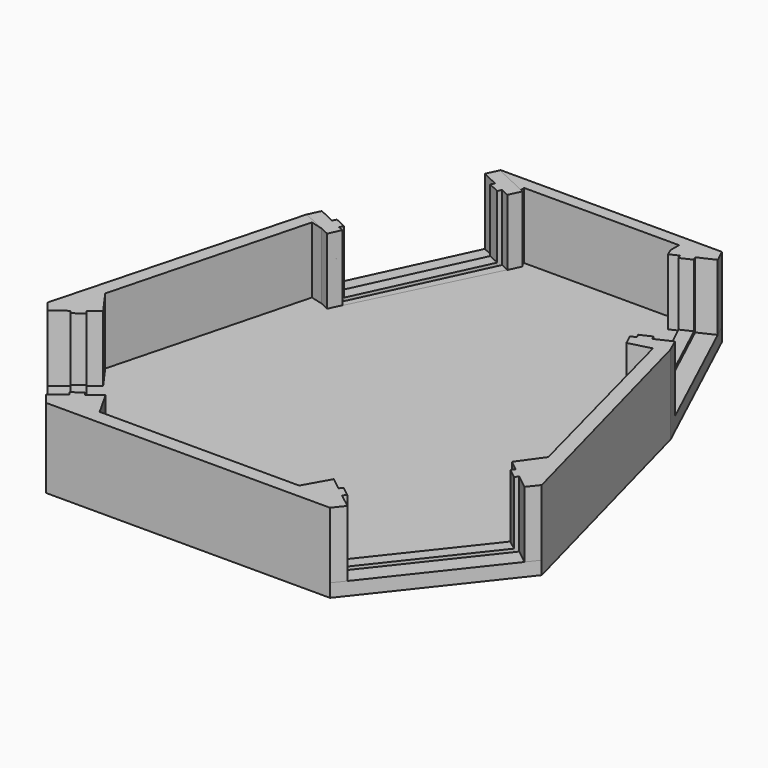
from build123d import *

# Parameters (mm, degrees)
F2_DEPTH  = 3
F4_DEPTH  = 0.7
F6_DEPTH  = 15
F7_DEPTH  = 0.7
F10_DEPTH = 15
F12_DEPTH = 3


with BuildPart() as f2:
    # F1 (on Top) → F2 (new body)
    with BuildSketch(Plane.XY):
        Polygon((25.0866528437, 0), (0, 0), (-25.0866528437, 0), (-41.3574559207, -34.8928498009), (-56.0353445751, -89.767503729), (-32.1974300433, -120), (0, -120), (32.1974300433, -120), (56.0353445751, -89.767503729), (41.3574559207, -34.8928498009), align=None)
    extrude(amount=-F2_DEPTH)

    # F3 (on face) → F4 (join)
    with BuildSketch(Plane.XY):
        Polygon((-33.371197317, -34.0930538801), (-20.5658639862, -6.6319279329), (-23.1035257899, -5.4485968), (-35.9088591207, -32.9097227472), align=None)
        Polygon((-50.2771969311, -90.448485161), (-31.5164486113, -114.2418523561), (-29.3177216098, -112.5081858447), (-48.0784699296, -88.7148186496), align=None)
        Polygon((20.5658639862, -6.6319279329), (33.371197317, -34.0930538801), (35.9088591207, -32.9097227472), (23.1035257899, -5.4485968), align=None)
        Polygon((29.3177216098, -112.5081858447), (31.5164486113, -114.2418523561), (50.2771969311, -90.448485161), (48.0784699296, -88.7148186496), align=None)
    extrude(amount=F4_DEPTH)

    # F5 (on face) → F6 (join)
    with BuildSketch(Plane.XY):
        Polygon((-23.1035257899, -5.4485968), (-20.5658639862, -6.6319279329), (-20.1643766376, -5.7709355352), (-18.2344874915, -6.6708576234), (-17.5556015009, -5.2149819182), (-17.5556015009, -2.7421381998), (0, -2.7421381998), (17.5556015009, -2.7421381998), (17.5556015009, -5.2149819182), (18.2344874915, -6.6708576234), (20.1643766376, -5.7709355352), (20.5658639862, -6.6319279329), (23.1035257899, -5.4485968), (22.7020384413, -4.5876044023), (26.4179003681, -2.8548695292), (25.0866528437, 0), (0, 0), (-25.0866528437, 0), (-26.4179003681, -2.8548695292), (-22.7020384413, -4.5876044023), align=None)
        Polygon((-33.7726846656, -34.9540462778), (-33.371197317, -34.0930538801), (-35.9088591207, -32.9097227472), (-36.3103464693, -33.7707151449), (-40.0262083962, -32.0379802717), (-41.3574559207, -34.8928498009), (-56.0353445751, -89.767503729), (-54.0849697497, -92.2410716057), (-50.8654052118, -89.7024884997), (-50.2771969311, -90.448485161), (-48.0784699296, -88.7148186496), (-48.6666782103, -87.9688219883), (-46.3434113852, -86.13695751), (-50.2389003724, -80.6826406293), (-38.6780583256, -36.5412120318), (-33.6958403856, -37.8460776983), (-32.6018529506, -35.5000140729), align=None)
        Polygon((-29.3177216098, -112.5081858447), (-31.5164486113, -114.2418523561), (-30.9282403307, -114.9878490173), (-34.1478048686, -117.5264321233), (-32.1974300433, -120), (0, -120), (32.1974300433, -120), (34.1478048686, -117.5264321233), (30.9282403307, -114.9878490173), (31.5164486113, -114.2418523561), (29.3177216098, -112.5081858447), (28.7295133292, -113.2541825059), (25.8780409714, -111.0058351069), (22.6252728403, -116.7735089854), (0, -116.7735089854), (-22.6252728403, -116.7735089854), (-25.8780409714, -111.0058351069), (-28.7295133292, -113.2541825059), align=None)
        Polygon((36.3103464693, -33.7707151449), (35.9088591207, -32.9097227472), (33.371197317, -34.0930538801), (33.7726846656, -34.9540462778), (32.6018529506, -35.5000140729), (33.6958403856, -37.8460776983), (38.6780583256, -36.5412120318), (50.2389003724, -80.6826406293), (46.3434113852, -86.13695751), (48.6666782103, -87.9688219883), (48.0784699296, -88.7148186496), (50.2771969311, -90.448485161), (50.8654052118, -89.7024884997), (54.0849697497, -92.2410716057), (56.0353445751, -89.767503729), (41.3574559207, -34.8928498009), (40.0262083962, -32.0379802717), align=None)
    extrude(amount=F6_DEPTH)


with BuildPart() as f7:
    # F3 (on face) → F7 (new body)
    with BuildSketch(Plane.XY):
        Polygon((-33.371197317, -34.0930538801), (-20.5658639862, -6.6319279329), (-23.1035257899, -5.4485968), (-35.9088591207, -32.9097227472), align=None)
    extrude(amount=F7_DEPTH)

    # F9 (on Top) → F10 (join)
    with BuildSketch(Plane.XY):
        Polygon((-33.371197317, -34.0930538801), (-35.9088591207, -32.9097227472), (-36.3103464693, -33.7707151449), (-40.0262083962, -32.0379802717), (-41.2940631814, -34.7569036329), (-33.8697077358, -38.218937434), (-32.6018529506, -35.5000140729), (-33.7726846656, -34.9540462778), align=None)
        Polygon((-20.5658639862, -6.6319279329), (-20.1643766376, -5.7709355352), (-18.2344874915, -6.6708576234), (-16.9666327063, -3.9519342623), (-25.1500455829, -0.1359461681), (-26.4179003681, -2.8548695292), (-22.7020384413, -4.5876044023), (-23.1035257899, -5.4485968), align=None)
    extrude(amount=F10_DEPTH)

    # F11 (on Top) → F12 (join)
    with BuildSketch(Plane.XY):
        Polygon((-41.2940631814, -34.7569036329), (-33.8697077358, -38.218937434), (-16.9666327063, -3.9519342623), (-25.1500455829, -0.1359461681), align=None)
    extrude(amount=-F12_DEPTH)


with BuildPart() as f7b:
    # F3 (on face) → F7, piece 2 (new body)
    with BuildSketch(Plane.XY):
        Polygon((-50.2771969311, -90.448485161), (-31.5164486113, -114.2418523561), (-29.3177216098, -112.5081858447), (-48.0784699296, -88.7148186496), align=None)
    extrude(amount=F7_DEPTH)


with BuildPart() as f7c:
    # F3 (on face) → F7, piece 3 (new body)
    with BuildSketch(Plane.XY):
        Polygon((20.5658639862, -6.6319279329), (33.371197317, -34.0930538801), (35.9088591207, -32.9097227472), (23.1035257899, -5.4485968), align=None)
    extrude(amount=F7_DEPTH)


with BuildPart() as f7d:
    # F3 (on face) → F7, piece 4 (new body)
    with BuildSketch(Plane.XY):
        Polygon((29.3177216098, -112.5081858447), (31.5164486113, -114.2418523561), (50.2771969311, -90.448485161), (48.0784699296, -88.7148186496), align=None)
    extrude(amount=F7_DEPTH)


solid = Compound([f2.part, f7.part])
